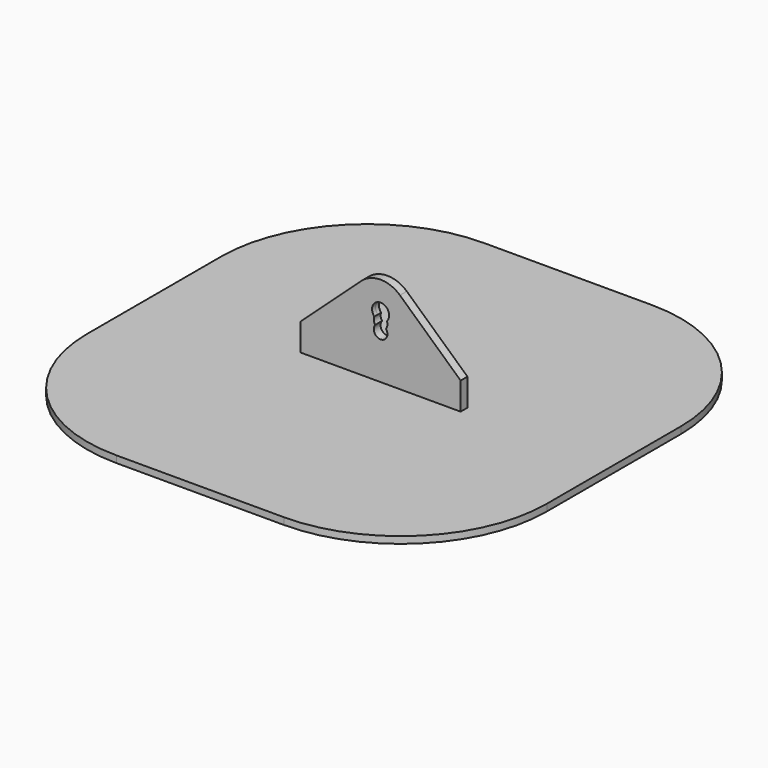
from build123d import *

# Parameters (mm, degrees)
F1_DEPTH = 2
F3_DEPTH = 2.5


with BuildPart() as f1:
    # F0 (on Top) → F1 (new body, symmetric)
    with BuildSketch(Plane.XY):
        with BuildLine():
            Line((49.1, 134.6), (-49.1, 134.6))
            ThreePointArc((-49.1, 134.6), (-109.5576297914, 109.5576297914), (-134.6, 49.1))
            Line((-134.6, 49.1), (-134.6, -49.1))
            ThreePointArc((-134.6, -49.1), (-109.5576297914, -109.5576297914), (-49.1, -134.6))
            Line((-49.1, -134.6), (49.1, -134.6))
            ThreePointArc((49.1, -134.6), (109.5576297914, -109.5576297914), (134.6, -49.1))
            Line((134.6, -49.1), (134.6, 49.1))
            ThreePointArc((134.6, 49.1), (109.5576297914, 109.5576297914), (49.1, 134.6))
        make_face()
    extrude(amount=F1_DEPTH, both=True)

    # F2 (on Front) → F3 (join, symmetric)
    with BuildSketch(Plane.XZ):
        with BuildLine():
            Line((-46.8736924231, 0), (0, 0))
            Line((0, 0), (46.8736924231, 0))
            Line((46.8736924231, 0), (46.8736924231, 18.0345661938))
            Line((46.8736924231, 18.0345661938), (11.3395565202, 50.4359355817))
            ThreePointArc((11.3395565202, 50.4359355817), (0, 54.829677236), (-11.3395565202, 50.4359355817))
            Line((-11.3395565202, 50.4359355817), (-46.8736924231, 18.0345661938))
            Line((-46.8736924231, 18.0345661938), (-46.8736924231, 0))
        make_face()
        with BuildLine():
            ThreePointArc((-3.666060556, 34.6), (-1.8261567868, 42.6545839116), (5, 38))
            ThreePointArc((5, 38), (4.6545839116, 36.1738432132), (3.666060556, 34.6))
            ThreePointArc((3.666060556, 34.6), (3.9156252517, 33.8172385748), (4, 33))
            ThreePointArc((4, 33), (3.7742546282, 31.6752351146), (3.1224989992, 30.5))
            ThreePointArc((3.1224989992, 30.5), (3.7742546282, 29.3247648854), (4, 28))
            ThreePointArc((4, 28), (-1.3247648854, 24.2257453718), (-3.1224989992, 30.5))
            ThreePointArc((-3.1224989992, 30.5), (-3.9653039239, 32.4742959088), (-3.666060556, 34.6))
        make_face(mode=Mode.SUBTRACT)
    extrude(amount=F3_DEPTH, both=True)


solid = f1.part
